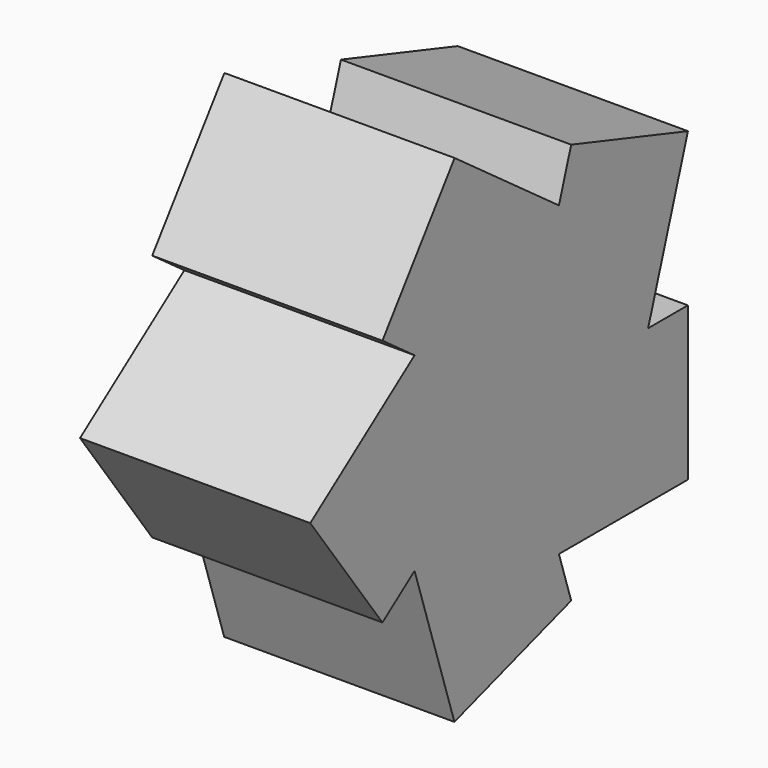
from build123d import *

# Parameters (mm, degrees)
F0_W     = 60
F0_H     = 55
F1_DEPTH = 40
F2_COUNT = 5


with BuildPart() as f1:
    # F0 (on Top) → F1 (new body)
    with BuildSketch(Plane.XY):
        with Locations((-30, 27.5)):
            Rectangle(F0_W, F0_H)
    extrude(amount=F1_DEPTH)

    # F2: F1 ×5 about axis
    f2_axis = Axis((-30, 0, 40), (-1, 0, 0))


with BuildPart() as f1_1:
    add(f1.part)
    for i in range(1, F2_COUNT):
        add(f1.part.rotate(f2_axis, i * 360 / F2_COUNT))


solid = f1_1.part
